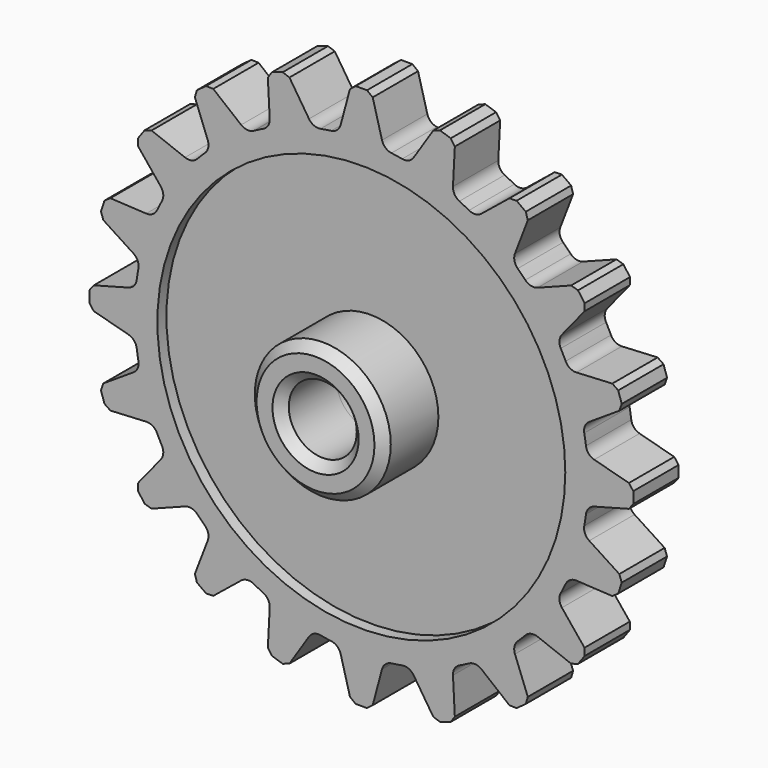
from build123d import *

# Parameters (mm, degrees)
F1_DEPTH        = 25
F3_DEPTH        = 25
F3_COPIES_COUNT = 20
F4_SIZE         = 2
F5_R            = 5
F6_R            = 90
F7_DEPTH        = 5
F8_R            = 30
F8_R_2          = 15
F9_DEPTH        = 30.265
F10_DEPTH       = 20.001
F11_SIZE        = 4


# Not quite as in the source:
# - a pattern or mirror of a feature is missing from the dataset's text; its kind, count and spacing are read off the source's solid


with BuildPart() as f1:
    # F0 (on Front) → F1 (new body)
    with BuildSketch(Plane.XZ):
        with BuildLine():
            ThreePointArc((-6.4939386792, 99.7889210305), (-68.3761878584, -72.9705209928), (100, 0))
            ThreePointArc((100, 0), (75.5292221679, 65.5388174955), (14.0932680257, 99.0019181448))
            ThreePointArc((14.0932680257, 99.0019181448), (3.8199862585, 99.9270118886), (-6.4939386792, 99.7889210305))
        make_face()
    extrude(amount=F1_DEPTH)

    # F2 (on face) → F3 (join)
    with BuildSketch(Plane.XZ.offset(25)):
        with BuildLine():
            ThreePointArc((-9.993, 99.4994469884), (0, 100), (9.993, 99.4994469884))
            Line((9.993, 99.4994469884), (4.5, 119.9996020744))
            Line((4.5, 119.9996020744), (-4.5, 119.9996020744))
            Line((-4.5, 119.9996020744), (-9.993, 99.4994469884))
        make_face()
    f3 = extrude(amount=-F3_DEPTH)

    # F3_copies: F3 ×20 about axis
    f3_copies_axis = Axis((0, 0, 0), (0, 1, 0))
    for i in range(1, F3_COPIES_COUNT):
        add(f3.rotate(f3_copies_axis, i * 360 / F3_COPIES_COUNT))

    # F4
    f4_edges = [f1.edges().sort_by_distance(p)[0] for p in [
        (-4.5, -12.5, 119.999602),
        (4.5, -12.5, 119.999602),
        (32.802162, -12.5, 115.51698),
        (-66.89342, -12.5, 99.726751),
        (-74.174573, -12.5, 94.436684),
        (-94.436684, -12.5, 74.174573),
        (-99.726751, -12.5, 66.89342),
        (-112.735827, -12.5, 41.361671),
        (-115.51698, -12.5, 32.802162),
        (-119.999602, -12.5, 4.5),
        (-119.999602, -12.5, -4.5),
        (-115.51698, -12.5, -32.802162),
        (-112.735827, -12.5, -41.361671),
        (-99.726751, -12.5, -66.89342),
        (-94.436684, -12.5, -74.174573),
        (-74.174573, -12.5, -94.436684),
        (-66.89342, -12.5, -99.726751),
        (-41.361671, -12.5, -112.735827),
        (-32.802162, -12.5, -115.51698),
        (-4.5, -12.5, -119.999602),
        (4.5, -12.5, -119.999602),
        (32.802162, -12.5, -115.51698),
        (41.361671, -12.5, -112.735827),
        (66.89342, -12.5, -99.726751),
        (74.174573, -12.5, -94.436684),
        (94.436684, -12.5, -74.174573),
        (99.726751, -12.5, -66.89342),
        (112.735827, -12.5, -41.361671),
        (115.51698, -12.5, -32.802162),
        (119.999602, -12.5, -4.5),
        (119.999602, -12.5, 4.5),
        (115.51698, -12.5, 32.802162),
        (112.735827, -12.5, 41.361671),
        (99.726751, -12.5, 66.89342),
        (94.436684, -12.5, 74.174573),
        (74.174573, -12.5, 94.436684),
        (66.89342, -12.5, 99.726751),
        (41.361671, -12.5, 112.735827),
        (-41.361671, -12.5, 112.735827),
        (-32.802162, -12.5, 115.51698),
    ]]
    chamfer(f4_edges, length=F4_SIZE)

    # F5
    f5_edges = [f1.edges().sort_by_distance(p)[0] for p in [
        (9.993, -12.5, 99.499447),
        (-9.993, -12.5, 99.499447),
        (21.243112, -12.5, 97.717604),
        (-21.243112, -12.5, 97.717604),
        (40.250928, -12.5, 91.541591),
        (50.399801, -12.5, 86.370482),
        (-40.250928, -12.5, 91.541591),
        (-50.399801, -12.5, 86.370482),
        (66.568814, -12.5, 74.623006),
        (74.623006, -12.5, 66.568814),
        (-66.568814, -12.5, 74.623006),
        (-74.623006, -12.5, 66.568814),
        (86.370482, -12.5, 50.399801),
        (91.541591, -12.5, 40.250928),
        (-86.370482, -12.5, 50.399801),
        (-91.541591, -12.5, 40.250928),
        (97.717604, -12.5, 21.243112),
        (99.499447, -12.5, 9.993),
        (-97.717604, -12.5, 21.243112),
        (-99.499447, -12.5, 9.993),
        (99.499447, -12.5, -9.993),
        (97.717604, -12.5, -21.243112),
        (-99.499447, -12.5, -9.993),
        (-97.717604, -12.5, -21.243112),
        (91.541591, -12.5, -40.250928),
        (86.370482, -12.5, -50.399801),
        (-91.541591, -12.5, -40.250928),
        (-86.370482, -12.5, -50.399801),
        (74.623006, -12.5, -66.568814),
        (66.568814, -12.5, -74.623006),
        (-74.623006, -12.5, -66.568814),
        (-66.568814, -12.5, -74.623006),
        (50.399801, -12.5, -86.370482),
        (40.250928, -12.5, -91.541591),
        (-50.399801, -12.5, -86.370482),
        (-40.250928, -12.5, -91.541591),
        (21.243112, -12.5, -97.717604),
        (9.993, -12.5, -99.499447),
        (-21.243112, -12.5, -97.717604),
        (-9.993, -12.5, -99.499447),
    ]]
    fillet(f5_edges, radius=F5_R)

    # F6 (on face) → F7 (cut)
    with BuildSketch(Plane.XZ.offset(25)):
        Circle(F6_R)
    extrude(amount=-F7_DEPTH, mode=Mode.SUBTRACT)

    # F8 (on face) → F9 (join)
    with BuildSketch(Plane.XZ.offset(20)):
        Circle(F8_R)
        Circle(F8_R_2, mode=Mode.SUBTRACT)
    extrude(amount=F9_DEPTH)

    # F10 (cut, through all): a face of the model
    f10_faces = [f1.faces().sort_by_distance(p)[0] for p in [
        (0, -20, 0),
    ]]
    extrude(f10_faces, amount=-F10_DEPTH, mode=Mode.SUBTRACT)

    # F11
    f11_edges = [f1.edges().sort_by_distance(p)[0] for p in [
        (-30, -50.265, 0),
        (-15, -50.265, 0),
    ]]
    chamfer(f11_edges, length=F11_SIZE)


solid = f1.part
